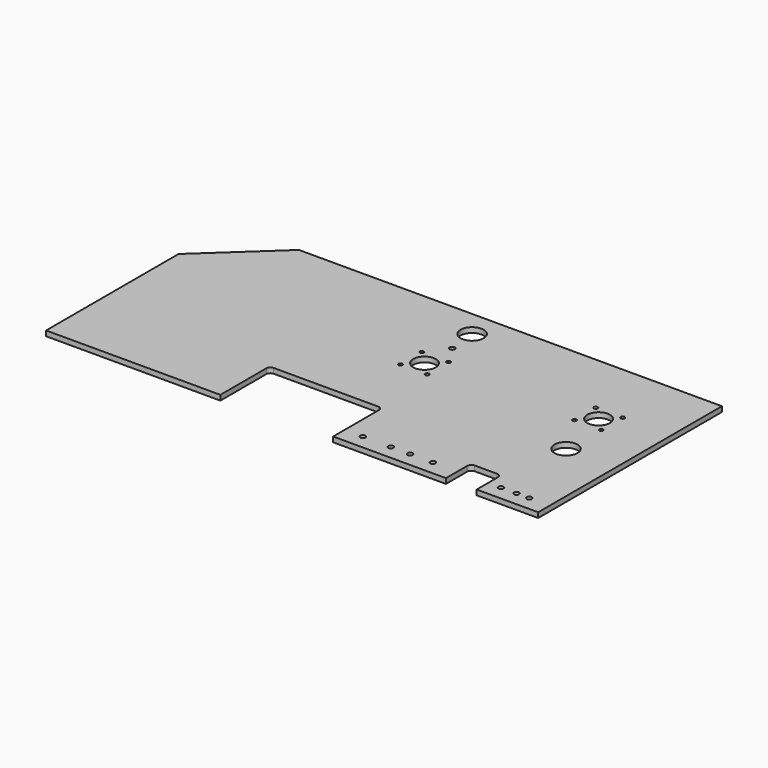
from build123d import *

# Parameters (mm, degrees)
F0_R     = 3.175
F0_R_2   = 3.1994548284
F0_R_3   = 14.2875
F0_R_4   = 2.413
F0_R_5   = 13.97
F1_DEPTH = 6.35
F2_R     = 5.08


# Not quite as in the source:
# - a length typed as a fraction of an inch, garbled in the dataset ("3 / 203.2 mm" for 3/8 in), is restored


with BuildPart() as f1:
    # F0 (on Top) → F1 (new body)
    with BuildSketch(Plane.XY):
        Polygon((570.0438245296, 36.7193375349), (46.0845124741, 36.7193375349), (-39.5561754704, -42.6550139801), (-39.5561754704, -247.7606624651), (176.3438245296, -247.7606624651), (176.3438245296, -171.5606624651), (316.0438245296, -171.5606624651), (316.0438245296, -247.7606624651), (455.7438245296, -247.7606624651), (455.7438245296, -209.6606624651), (493.8438245296, -209.6606624651), (493.8438245296, -247.7606624651), (570.0438245296, -247.7606624651), align=None)
        with Locations((338.6971652508, -229.9806624651)):
            Circle(F0_R, mode=Mode.SUBTRACT)
        with Locations((373.4027445316, -229.9806624651)):
            Circle(F0_R, mode=Mode.SUBTRACT)
        with Locations((397.1410393715, -229.9806624651)):
            Circle(F0_R, mode=Mode.SUBTRACT)
        with Locations((425.3449738026, -229.9806624651)):
            Circle(F0_R_2, mode=Mode.SUBTRACT)
        with Locations((509.7217559814, -229.9806624651)):
            Circle(F0_R_2, mode=Mode.SUBTRACT)
        with Locations((529.0057063103, -229.9806624651)):
            Circle(F0_R_2, mode=Mode.SUBTRACT)
        with Locations((544.7416305542, -229.9806624651)):
            Circle(F0_R_2, mode=Mode.SUBTRACT)
        with Locations((508.030295372, -127.1675527096)):
            Circle(F0_R_3, mode=Mode.SUBTRACT)
        with Locations((272.5348336594, -89.2630653484)):
            Circle(F0_R_4, mode=Mode.SUBTRACT)
        with Locations((305.7173030479, -89.2630653484)):
            Circle(F0_R_4, mode=Mode.SUBTRACT)
        with Locations((289.1260683537, -72.6718306541)):
            Circle(F0_R_5, mode=Mode.SUBTRACT)
        with Locations((272.5348336594, -56.0805959599)):
            Circle(F0_R_4, mode=Mode.SUBTRACT)
        with Locations((305.7173030479, -56.0805959599)):
            Circle(F0_R_4, mode=Mode.SUBTRACT)
        with Locations((476.8743677037, -75.141350369)):
            Circle(F0_R_4, mode=Mode.SUBTRACT)
        with Locations((510.0568370922, -75.141350369)):
            Circle(F0_R_4, mode=Mode.SUBTRACT)
        with Locations((493.4656023979, -58.5501156747)):
            Circle(F0_R_5, mode=Mode.SUBTRACT)
        with Locations((476.8743677037, -41.9588809805)):
            Circle(F0_R_4, mode=Mode.SUBTRACT)
        with Locations((510.0568370922, -41.9588809805)):
            Circle(F0_R_4, mode=Mode.SUBTRACT)
        with Locations((290.5568880873, -31.5565178133)):
            Circle(F0_R, mode=Mode.SUBTRACT)
        with Locations((286.8396043777, 3.9247339591)):
            Circle(F0_R_3, mode=Mode.SUBTRACT)
    extrude(amount=F1_DEPTH)

    # F2
    f2_edges = [f1.edges().sort_by_distance(p)[0] for p in [
        (176.343825, -171.560662, 3.175),
        (316.043825, -171.560662, 3.175),
        (455.743825, -209.660662, 3.175),
        (493.843825, -209.660662, 3.175),
    ]]
    fillet(f2_edges, radius=F2_R)


solid = f1.part
